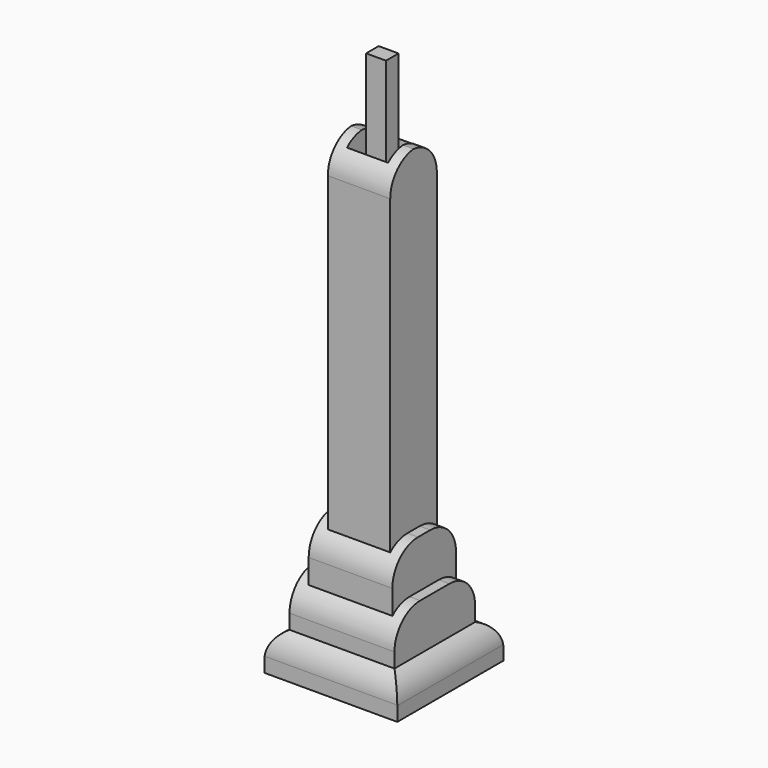
from build123d import *

# Parameters (mm, degrees)
F0_W         = 100.2616621554
F0_H         = 96.2751097977
F1_DEPTH     = 81.788
F0_W_2       = 127
F0_H_2       = 127
F2_DEPTH     = 3.81
F3_DEPTH     = 33.274
F4_W         = 79.9416621554
F4_H         = 75.9551097977
F4_W_2       = 59.6216621554
F4_H_2       = 55.6351097977
F5_DEPTH     = 45.974
F4_W_3       = 39.3016621554
F4_H_3       = 35.3151097977
F6_DEPTH     = 366.268
F4_W_4       = 18.9816621554
F4_H_4       = 14.9951097977
F7_DEPTH     = 436.88
F8_T1_DEPTH  = 244.5410255238
F8_T3_DEPTH  = 271.366739111
F8_T5_DEPTH  = 241.9714995397
F8_T7_DEPTH  = 260.9845639802
F8_T12_DEPTH = 253.5642233661
F8_T17_DEPTH = 253.5642233661
F8_T22_DEPTH = 253.5642233661
F8_T27_DEPTH = 233.2442233661
F8_T32_DEPTH = 233.2442233661
F8_T37_DEPTH = 233.2442233661
F8_T42_DEPTH = 212.9242233661
F8_T47_DEPTH = 212.9242233661
F8_T52_DEPTH = 212.9242233661
F8_T57_DEPTH = 253.5642233661
F8_T62_DEPTH = 253.5642233661
F8_T67_DEPTH = 253.5642233661
F8_T72_DEPTH = 233.2442233661
F8_T77_DEPTH = 233.2442233661
F8_T82_DEPTH = 233.2442233661
F8_T87_DEPTH = 212.9242233661
F8_T92_DEPTH = 212.9242233661
F8_T97_DEPTH = 212.9242233661


# Not quite as in the source:
# - a fillet or chamfer that OpenCascade refuses, or shapes differently, is made with other operations: its cross-section is extruded or revolved along the edge and cut away or added


with BuildPart() as f1:
    # F0 (on Top) → F1 (new body)
    with BuildSketch(Plane.XY):
        with Locations((-10.751856491, -7.9730954021)):
            Rectangle(F0_W, F0_H)
    extrude(amount=F1_DEPTH)

    # F0 (on Top) → F2 (join)
    with BuildSketch(Plane.XY):
        with Locations((-13.1437878911, -2.989910543)):
            Rectangle(F0_W_2, F0_H_2)
        with Locations((-10.751856491, -7.9730954021)):
            Rectangle(F0_W, F0_H, mode=Mode.SUBTRACT)
    extrude(amount=F2_DEPTH)

    # F3 (add): a face of the model
    f3_faces = [f1.faces().sort_by_distance(p)[0] for p in [
        (-13.1437878911, 58.7140382328, 3.81),
    ]]
    extrude(f3_faces, amount=F3_DEPTH)

    # F4 (on face) → F5 (join)
    with BuildSketch(Plane.XY.offset(81.788)):
        with Locations((-10.751856491, -7.9730954021)):
            Rectangle(F4_W, F4_H)
        with Locations((-10.751856491, -7.9730954021)):
            Rectangle(F4_W_2, F4_H_2, mode=Mode.SUBTRACT)
    extrude(amount=F5_DEPTH)

    # F4 (on face) → F6 (join)
    with BuildSketch(Plane.XY.offset(81.788)):
        with Locations((-10.751856491, -7.9730954021)):
            Rectangle(F4_W_2, F4_H_2)
        with Locations((-10.751856491, -7.9730954021)):
            Rectangle(F4_W_3, F4_H_3, mode=Mode.SUBTRACT)
    extrude(amount=F6_DEPTH)

    # F4 (on face) → F7 (join)
    with BuildSketch(Plane.XY.offset(81.788)):
        with Locations((-10.751856491, -7.9730954021)):
            Rectangle(F4_W_4, F4_H_4)
    extrude(amount=F7_DEPTH)

    # F8: fillet of radius 30.6605122421 on 10 edges, made by hand

    # F8_s2 → F8_t1 (cut)
    with BuildSketch(Plane.XZ.offset(-119.280602219)):
        with BuildLine():
            ThreePointArc((39.3789745867, 37.084), (47.4766852386, 26.5482219124), (50.3562121089, 13.5757948952))
            Line((50.3562121089, 13.5757948952), (50.3562121089, 37.084))
            Line((50.3562121089, 37.084), (39.3789745867, 37.084))
        make_face()
    extrude(amount=F8_T1_DEPTH, mode=Mode.SUBTRACT)

    # F8_s4 → F8_t3 (cut)
    with BuildSketch(Plane.YZ.offset(-148.8271574466)):
        with BuildLine():
            ThreePointArc((40.1644594967, 37.084), (54.9127632198, 25.8714482594), (60.510089457, 8.2106521778))
            Line((60.510089457, 8.2106521778), (60.510089457, 37.084))
            Line((60.510089457, 37.084), (40.1644594967, 37.084))
        make_face()
    extrude(amount=F8_T3_DEPTH, mode=Mode.SUBTRACT)

    # F8_s6 → F8_t5 (cut)
    with BuildSketch(Plane.YZ.offset(-134.129537661)):
        with BuildLine():
            ThreePointArc((-56.110650301, 37.084), (-63.7748861852, 26.70384762), (-66.489910543, 14.0897000921))
            Line((-66.489910543, 14.0897000921), (-66.489910543, 37.084))
            Line((-66.489910543, 37.084), (-56.110650301, 37.084))
        make_face()
    extrude(amount=F8_T5_DEPTH, mode=Mode.SUBTRACT)

    # F8_s8 → F8_t7 (cut)
    with BuildSketch(Plane.XZ.offset(-127.5023714471)):
        with BuildLine():
            ThreePointArc((-60.8826875687, 37.084), (-72.4113914777, 25.831272763), (-76.6437878911, 10.287087204))
            Line((-76.6437878911, 10.287087204), (-76.6437878911, 37.084))
            Line((-76.6437878911, 37.084), (-60.8826875687, 37.084))
        make_face()
    extrude(amount=F8_T7_DEPTH, mode=Mode.SUBTRACT)


with BuildPart() as f8_tool10:
    # F8_s11 → F8_t12 (new body)
    with BuildSketch(Plane.YZ.offset(-137.533968174)):
        with BuildLine():
            ThreePointArc((-25.4501380588, 81.788), (-47.1303941799, 72.8077438789), (-56.110650301, 51.1274877579))
            Line((-56.110650301, 51.1274877579), (-56.110650301, 81.788))
            Line((-56.110650301, 81.788), (-25.4501380588, 81.788))
        make_face()
    extrude(amount=F8_T12_DEPTH)

    split(bisect_by=Plane.YZ.offset(-50.7226875687), keep=Keep.BOTTOM)


with BuildPart() as f1_1:
    add(f1.part)

    # F8_t9: cut F8_tool10
    add(f8_tool10.part, mode=Mode.SUBTRACT)


with BuildPart() as f8_tool15:
    # F8_s16 → F8_t17 (new body)
    with BuildSketch(Plane.YZ.offset(-137.533968174)):
        with BuildLine():
            ThreePointArc((-25.4501380588, 81.788), (-47.1303941799, 72.8077438789), (-56.110650301, 51.1274877579))
            Line((-56.110650301, 51.1274877579), (-56.110650301, 81.788))
            Line((-56.110650301, 81.788), (-25.4501380588, 81.788))
        make_face()
    extrude(amount=F8_T17_DEPTH)

    split(bisect_by=Plane.XZ.offset(45.950650301), keep=Keep.TOP)


with BuildPart() as f1_2:
    add(f1_1.part)

    # F8_t14: cut F8_tool15
    add(f8_tool15.part, mode=Mode.SUBTRACT)


with BuildPart() as f8_tool20:
    # F8_s21 → F8_t22 (new body)
    with BuildSketch(Plane.YZ.offset(-137.533968174)):
        with BuildLine():
            ThreePointArc((-25.4501380588, 81.788), (-47.1303941799, 72.8077438789), (-56.110650301, 51.1274877579))
            Line((-56.110650301, 51.1274877579), (-56.110650301, 81.788))
            Line((-56.110650301, 81.788), (-25.4501380588, 81.788))
        make_face()
    extrude(amount=F8_T22_DEPTH)

    split(bisect_by=Plane.YZ.offset(29.2189745867), keep=Keep.TOP)


with BuildPart() as f1_3:
    add(f1_2.part)

    # F8_t19: cut F8_tool20
    add(f8_tool20.part, mode=Mode.SUBTRACT)


with BuildPart() as f8_tool25:
    # F8_s26 → F8_t27 (new body)
    with BuildSketch(Plane.YZ.offset(-127.373968174)):
        with BuildLine():
            ThreePointArc((-45.950650301, 97.1014877579), (-36.9703941799, 118.7817438789), (-15.2901380588, 127.762))
            Line((-15.2901380588, 127.762), (-45.950650301, 127.762))
            Line((-45.950650301, 127.762), (-45.950650301, 97.1014877579))
        make_face()
    extrude(amount=F8_T27_DEPTH)

    split(bisect_by=Plane.XZ.offset(35.790650301), keep=Keep.TOP)


with BuildPart() as f1_4:
    add(f1_3.part)

    # F8_t24: cut F8_tool25
    add(f8_tool25.part, mode=Mode.SUBTRACT)


with BuildPart() as f8_tool30:
    # F8_s31 → F8_t32 (new body)
    with BuildSketch(Plane.YZ.offset(-127.373968174)):
        with BuildLine():
            ThreePointArc((-45.950650301, 97.1014877579), (-36.9703941799, 118.7817438789), (-15.2901380588, 127.762))
            Line((-15.2901380588, 127.762), (-45.950650301, 127.762))
            Line((-45.950650301, 127.762), (-45.950650301, 97.1014877579))
        make_face()
    extrude(amount=F8_T32_DEPTH)

    split(bisect_by=Plane.YZ.offset(-40.5626875687), keep=Keep.BOTTOM)


with BuildPart() as f1_5:
    add(f1_4.part)

    # F8_t29: cut F8_tool30
    add(f8_tool30.part, mode=Mode.SUBTRACT)


with BuildPart() as f8_tool35:
    # F8_s36 → F8_t37 (new body)
    with BuildSketch(Plane.YZ.offset(-127.373968174)):
        with BuildLine():
            ThreePointArc((-45.950650301, 97.1014877579), (-36.9703941799, 118.7817438789), (-15.2901380588, 127.762))
            Line((-15.2901380588, 127.762), (-45.950650301, 127.762))
            Line((-45.950650301, 127.762), (-45.950650301, 97.1014877579))
        make_face()
    extrude(amount=F8_T37_DEPTH)

    split(bisect_by=Plane.YZ.offset(19.0589745867), keep=Keep.TOP)


with BuildPart() as f1_6:
    add(f1_5.part)

    # F8_t34: cut F8_tool35
    add(f8_tool35.part, mode=Mode.SUBTRACT)


with BuildPart() as f8_tool40:
    # F8_s41 → F8_t42 (new body)
    with BuildSketch(Plane.YZ.offset(-117.213968174)):
        with BuildLine():
            ThreePointArc((-35.790650301, 417.3954877579), (-26.8103941799, 439.0757438789), (-5.1301380588, 448.056))
            Line((-5.1301380588, 448.056), (-35.790650301, 448.056))
            Line((-35.790650301, 448.056), (-35.790650301, 417.3954877579))
        make_face()
    extrude(amount=F8_T42_DEPTH)

    split(bisect_by=Plane.XZ.offset(15.470650301), keep=Keep.TOP)


with BuildPart() as f1_7:
    add(f1_6.part)

    # F8_t39: cut F8_tool40
    add(f8_tool40.part, mode=Mode.SUBTRACT)


with BuildPart() as f8_tool45:
    # F8_s46 → F8_t47 (new body)
    with BuildSketch(Plane.YZ.offset(-117.213968174)):
        with BuildLine():
            ThreePointArc((-35.790650301, 417.3954877579), (-26.8103941799, 439.0757438789), (-5.1301380588, 448.056))
            Line((-5.1301380588, 448.056), (-35.790650301, 448.056))
            Line((-35.790650301, 448.056), (-35.790650301, 417.3954877579))
        make_face()
    extrude(amount=F8_T47_DEPTH)

    split(bisect_by=Plane.YZ.offset(-20.2426875687), keep=Keep.BOTTOM)


with BuildPart() as f1_8:
    add(f1_7.part)

    # F8_t44: cut F8_tool45
    add(f8_tool45.part, mode=Mode.SUBTRACT)


with BuildPart() as f8_tool50:
    # F8_s51 → F8_t52 (new body)
    with BuildSketch(Plane.YZ.offset(-117.213968174)):
        with BuildLine():
            ThreePointArc((-35.790650301, 417.3954877579), (-26.8103941799, 439.0757438789), (-5.1301380588, 448.056))
            Line((-5.1301380588, 448.056), (-35.790650301, 448.056))
            Line((-35.790650301, 448.056), (-35.790650301, 417.3954877579))
        make_face()
    extrude(amount=F8_T52_DEPTH)

    split(bisect_by=Plane.YZ.offset(-1.2610254133), keep=Keep.TOP)


with BuildPart() as f1_9:
    add(f1_8.part)

    # F8_t49: cut F8_tool50
    add(f8_tool50.part, mode=Mode.SUBTRACT)


with BuildPart() as f8_tool55:
    # F8_s56 → F8_t57 (new body)
    with BuildSketch(Plane.YZ.offset(116.0302551921)):
        with BuildLine():
            ThreePointArc((40.1644594967, 51.1274877579), (31.1842033757, 72.8077438789), (9.5039472546, 81.788))
            Line((9.5039472546, 81.788), (40.1644594967, 81.788))
            Line((40.1644594967, 81.788), (40.1644594967, 51.1274877579))
        make_face()
    extrude(amount=-F8_T57_DEPTH)

    split(bisect_by=Plane.XZ.offset(-30.0044594967), keep=Keep.BOTTOM)


with BuildPart() as f1_10:
    add(f1_9.part)

    # F8_t54: cut F8_tool55
    add(f8_tool55.part, mode=Mode.SUBTRACT)


with BuildPart() as f8_tool60:
    # F8_s61 → F8_t62 (new body)
    with BuildSketch(Plane.YZ.offset(116.0302551921)):
        with BuildLine():
            ThreePointArc((40.1644594967, 51.1274877579), (31.1842033757, 72.8077438789), (9.5039472546, 81.788))
            Line((9.5039472546, 81.788), (40.1644594967, 81.788))
            Line((40.1644594967, 81.788), (40.1644594967, 51.1274877579))
        make_face()
    extrude(amount=-F8_T62_DEPTH)

    split(bisect_by=Plane.YZ.offset(29.2189745867), keep=Keep.TOP)


with BuildPart() as f1_11:
    add(f1_10.part)

    # F8_t59: cut F8_tool60
    add(f8_tool60.part, mode=Mode.SUBTRACT)


with BuildPart() as f8_tool65:
    # F8_s66 → F8_t67 (new body)
    with BuildSketch(Plane.YZ.offset(116.0302551921)):
        with BuildLine():
            ThreePointArc((40.1644594967, 51.1274877579), (31.1842033757, 72.8077438789), (9.5039472546, 81.788))
            Line((9.5039472546, 81.788), (40.1644594967, 81.788))
            Line((40.1644594967, 81.788), (40.1644594967, 51.1274877579))
        make_face()
    extrude(amount=-F8_T67_DEPTH)

    split(bisect_by=Plane.YZ.offset(-50.7226875687), keep=Keep.BOTTOM)


with BuildPart() as f1_12:
    add(f1_11.part)

    # F8_t64: cut F8_tool65
    add(f8_tool65.part, mode=Mode.SUBTRACT)


with BuildPart() as f8_tool70:
    # F8_s71 → F8_t72 (new body)
    with BuildSketch(Plane.YZ.offset(105.8702551921)):
        with BuildLine():
            ThreePointArc((30.0044594967, 97.1014877579), (21.0242033757, 118.7817438789), (-0.6560527454, 127.762))
            Line((-0.6560527454, 127.762), (30.0044594967, 127.762))
            Line((30.0044594967, 127.762), (30.0044594967, 97.1014877579))
        make_face()
    extrude(amount=-F8_T72_DEPTH)

    split(bisect_by=Plane.XZ.offset(-19.8444594967), keep=Keep.BOTTOM)


with BuildPart() as f1_13:
    add(f1_12.part)

    # F8_t69: cut F8_tool70
    add(f8_tool70.part, mode=Mode.SUBTRACT)


with BuildPart() as f8_tool75:
    # F8_s76 → F8_t77 (new body)
    with BuildSketch(Plane.YZ.offset(105.8702551921)):
        with BuildLine():
            ThreePointArc((30.0044594967, 97.1014877579), (21.0242033757, 118.7817438789), (-0.6560527454, 127.762))
            Line((-0.6560527454, 127.762), (30.0044594967, 127.762))
            Line((30.0044594967, 127.762), (30.0044594967, 97.1014877579))
        make_face()
    extrude(amount=-F8_T77_DEPTH)

    split(bisect_by=Plane.YZ.offset(19.0589745867), keep=Keep.TOP)


with BuildPart() as f1_14:
    add(f1_13.part)

    # F8_t74: cut F8_tool75
    add(f8_tool75.part, mode=Mode.SUBTRACT)


with BuildPart() as f8_tool80:
    # F8_s81 → F8_t82 (new body)
    with BuildSketch(Plane.YZ.offset(105.8702551921)):
        with BuildLine():
            ThreePointArc((30.0044594967, 97.1014877579), (21.0242033757, 118.7817438789), (-0.6560527454, 127.762))
            Line((-0.6560527454, 127.762), (30.0044594967, 127.762))
            Line((30.0044594967, 127.762), (30.0044594967, 97.1014877579))
        make_face()
    extrude(amount=-F8_T82_DEPTH)

    split(bisect_by=Plane.YZ.offset(-40.5626875687), keep=Keep.BOTTOM)


with BuildPart() as f1_15:
    add(f1_14.part)

    # F8_t79: cut F8_tool80
    add(f8_tool80.part, mode=Mode.SUBTRACT)


with BuildPart() as f8_tool85:
    # F8_s86 → F8_t87 (new body)
    with BuildSketch(Plane.YZ.offset(95.7102551921)):
        with BuildLine():
            ThreePointArc((19.8444594967, 417.3954877579), (10.8642033757, 439.0757438789), (-10.8160527454, 448.056))
            Line((-10.8160527454, 448.056), (19.8444594967, 448.056))
            Line((19.8444594967, 448.056), (19.8444594967, 417.3954877579))
        make_face()
    extrude(amount=-F8_T87_DEPTH)

    split(bisect_by=Plane.XZ.offset(0.4755405033), keep=Keep.BOTTOM)


with BuildPart() as f1_16:
    add(f1_15.part)

    # F8_t84: cut F8_tool85
    add(f8_tool85.part, mode=Mode.SUBTRACT)


with BuildPart() as f8_tool90:
    # F8_s91 → F8_t92 (new body)
    with BuildSketch(Plane.YZ.offset(95.7102551921)):
        with BuildLine():
            ThreePointArc((19.8444594967, 417.3954877579), (10.8642033757, 439.0757438789), (-10.8160527454, 448.056))
            Line((-10.8160527454, 448.056), (19.8444594967, 448.056))
            Line((19.8444594967, 448.056), (19.8444594967, 417.3954877579))
        make_face()
    extrude(amount=-F8_T92_DEPTH)

    split(bisect_by=Plane.YZ.offset(-1.2610254133), keep=Keep.TOP)


with BuildPart() as f1_17:
    add(f1_16.part)

    # F8_t89: cut F8_tool90
    add(f8_tool90.part, mode=Mode.SUBTRACT)


with BuildPart() as f8_tool95:
    # F8_s96 → F8_t97 (new body)
    with BuildSketch(Plane.YZ.offset(95.7102551921)):
        with BuildLine():
            ThreePointArc((19.8444594967, 417.3954877579), (10.8642033757, 439.0757438789), (-10.8160527454, 448.056))
            Line((-10.8160527454, 448.056), (19.8444594967, 448.056))
            Line((19.8444594967, 448.056), (19.8444594967, 417.3954877579))
        make_face()
    extrude(amount=-F8_T97_DEPTH)

    split(bisect_by=Plane.YZ.offset(-20.2426875687), keep=Keep.BOTTOM)


with BuildPart() as f1_18:
    add(f1_17.part)

    # F8_t94: cut F8_tool95
    add(f8_tool95.part, mode=Mode.SUBTRACT)


solid = f1_18.part
